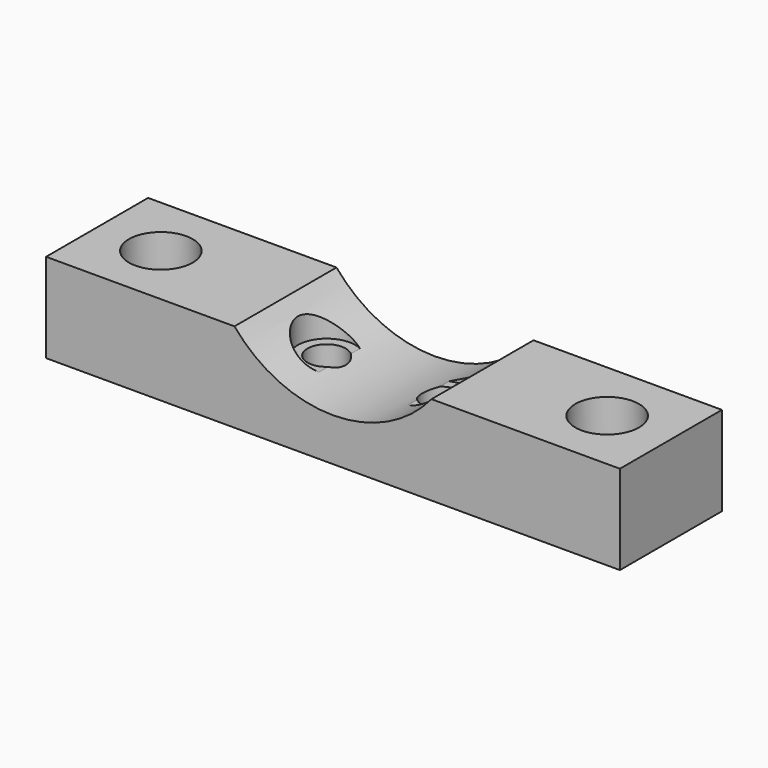
from build123d import *

# Parameters (mm, degrees)
F0_R     = 1.5
F0_R_2   = 1.75
F1_DEPTH = 7
F2_R     = 2.5
F2_R_2   = 1.75
F2_R_3   = 2.25
F2_R_4   = 1.5
F3_DEPTH = 3
F5_DEPTH = 25


with BuildPart() as f1:
    # F0 (on Top) → F1 (new body)
    with BuildSketch(Plane.XY):
        Polygon((22.5, 0), (22.5, 5), (-22.5, 5), (-22.5, 0), (-22.5, -5), (22.5, -5), align=None)
        with BuildLine():
            ThreePointArc((-15.75, 0), (-17.5, -1.75), (-19.25, 0))
            ThreePointArc((-19.25, 0), (-17.5, 1.75), (-15.75, 0))
        make_face(mode=Mode.SUBTRACT)
        with Locations((-4.5, 0)):
            Circle(F0_R, mode=Mode.SUBTRACT)
        with Locations((4.5, 0)):
            Circle(F0_R, mode=Mode.SUBTRACT)
        with Locations((17.5, 0)):
            Circle(F0_R_2, mode=Mode.SUBTRACT)
    extrude(amount=F1_DEPTH)

    # F2 (on face) → F3 (cut)
    with BuildSketch(Plane.XY.offset(7)):
        with Locations((-17.5, 0)):
            Circle(F2_R)
        with Locations((-17.5, 0)):
            Circle(F2_R_2, mode=Mode.SUBTRACT)
        with Locations((-4.5, 0)):
            Circle(F2_R_3)
        with Locations((-4.5, 0)):
            Circle(F2_R_4, mode=Mode.SUBTRACT)
        with Locations((4.5, 0)):
            Circle(F2_R_3)
        with Locations((4.5, 0)):
            Circle(F2_R_4, mode=Mode.SUBTRACT)
        with Locations((17.5, 0)):
            Circle(F2_R)
        with Locations((17.5, 0)):
            Circle(F2_R_2, mode=Mode.SUBTRACT)
    extrude(amount=-F3_DEPTH, mode=Mode.SUBTRACT)

    # F4 (on face) → F5 (cut)
    with BuildSketch(Plane(origin=(0, 5, 0), x_dir=(-1, 0, 0), z_dir=(0, 1, 0))):
        with BuildLine():
            Line((0, 7), (-7.72596329, 7))
            ThreePointArc((-7.72596329, 7), (0, 3.3733951654), (7.72596329, 7))
            Line((7.72596329, 7), (0, 7))
        make_face()
    extrude(amount=-F5_DEPTH, mode=Mode.SUBTRACT)


solid = f1.part
